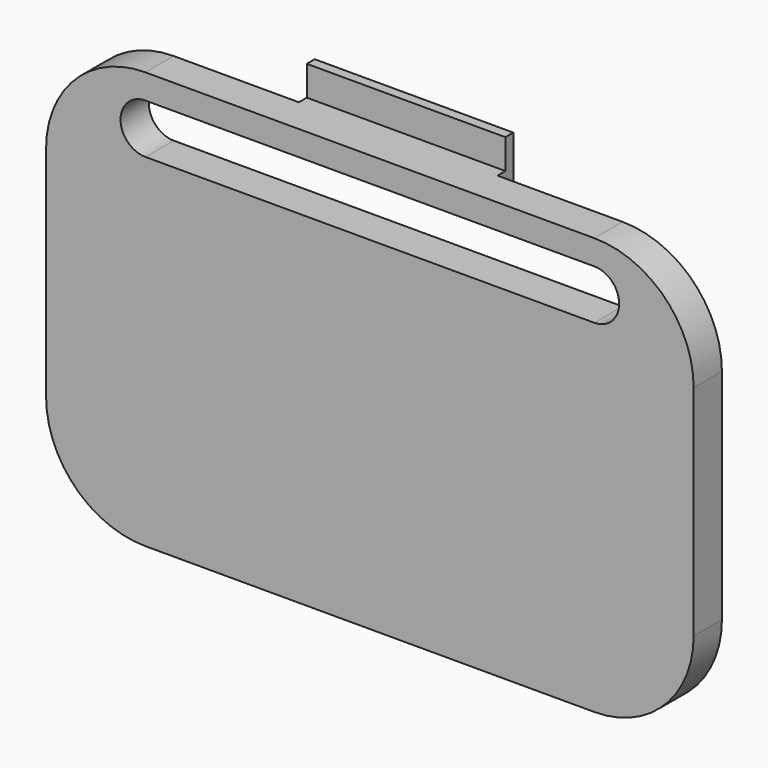
from build123d import *

# Parameters (mm, degrees)
F1_DEPTH  = 2.2606
F2_W      = 25.9304894134
F2_H      = 7.9375
F3_DEPTH  = 0.396875
F4_W      = 14.351
F4_H      = 1.778
F5_DEPTH  = 1.27
F6_SIZE   = 0.79375
F10_DEPTH = 2.2606
F12_DEPTH = 6.35
F13_W     = 0.635
F13_H     = 1.778
F14_DEPTH = 27.8775


# Not quite as in the source:
# - a feature names something its author has since deleted; it is built from what else it names


with BuildPart() as f1:
    # F0 (on Front) → F1 (new body)
    with BuildSketch(Plane.XZ):
        with BuildLine():
            ThreePointArc((0, 6.35), (1.8598719395, 1.8598719395), (6.35, 0))
            Line((6.35, 0), (35.052, 0))
            ThreePointArc((35.052, 0), (39.5421280605, 1.8598719395), (41.402, 6.35))
            Line((41.402, 6.35), (41.402, 20.32))
            ThreePointArc((41.402, 20.32), (39.5421280605, 24.8101280605), (35.052, 26.67))
            Line((35.052, 26.67), (6.35, 26.67))
            ThreePointArc((6.35, 26.67), (1.8598719395, 24.8101280605), (0, 20.32))
            Line((0, 20.32), (0, 6.35))
        make_face()
    extrude(amount=-F1_DEPTH)

    # F2 (on face) → F3 (cut)
    with BuildSketch(Plane(origin=(0, 2.2606, 0), x_dir=(-1, 0, 0), z_dir=(0, 1, 0))):
        with Locations((-20.4992552933, 10.57275)):
            Rectangle(F2_W, F2_H)
    extrude(amount=-F3_DEPTH, mode=Mode.SUBTRACT)

    # F4 (on face) → F5 (join)
    with BuildSketch(Plane(origin=(0, 2.2606, 0), x_dir=(-1, 0, 0), z_dir=(0, 1, 0))):
        with Locations((-20.701, -0.889)):
            Rectangle(F4_W, F4_H)
        Polygon((-21.209, 2.38125), (-26.8605, 2.38125), (-26.8605, 6.2865), (-27.8765, 6.2865), (-27.8765, 0), (-13.5255, 0), (-13.5255, 6.2865), (-14.5415, 6.2865), (-14.5415, 2.38125), (-20.193, 2.38125), (-20.193, 6.2865), (-21.209, 6.2865), align=None)
    extrude(amount=F5_DEPTH)

    # F6
    f6_edges = [f1.edges().sort_by_distance(p)[0] for p in [
        (27.3685, 3.5306, 6.2865),
        (20.701, 3.5306, 6.2865),
        (14.0335, 3.5306, 6.2865),
    ]]
    chamfer(f6_edges, length=F6_SIZE)

    # F9 (on Front) → F10 (cut, through all)
    with BuildSketch(Plane.XZ):
        with BuildLine():
            Line((6.35, 21.9075), (35.052, 21.9075))
            ThreePointArc((35.052, 21.9075), (36.6395, 23.495), (35.052, 25.0825))
            Line((35.052, 25.0825), (6.35, 25.0825))
            ThreePointArc((6.35, 25.0825), (4.7625, 23.495), (6.35, 21.9075))
        make_face()
    extrude(amount=-F10_DEPTH, mode=Mode.SUBTRACT)

    # F11 (on face) → F12 (join, symmetric)
    with BuildSketch(Plane.YZ.offset(20.701)):
        with BuildLine():
            Line((2.2606, 26.67), (2.2606, 25.1591298729))
            Line((2.2606, 25.1591298729), (2.8956, 25.1591298729))
            ThreePointArc((2.8956, 25.1591298729), (3.3446128061, 25.3451170669), (3.5306, 25.7941298729))
            Line((3.5306, 25.7941298729), (3.5306, 26.67))
            Line((3.5306, 26.67), (3.5306, 28.575))
            Line((3.5306, 28.575), (2.8956, 28.575))
            Line((2.8956, 28.575), (2.8956, 26.67))
            Line((2.8956, 26.67), (2.2606, 26.67))
        make_face()
    extrude(amount=F12_DEPTH, both=True)

    # F13 (on face) → F14 (cut, through all)
    with BuildSketch(Plane(origin=(13.5255, 0, 0), x_dir=(0, -1, 0), z_dir=(-1, 0, 0))):
        with Locations((-2.5781, -0.889)):
            Rectangle(F13_W, F13_H)
    extrude(amount=-F14_DEPTH, mode=Mode.SUBTRACT)


solid = f1.part
